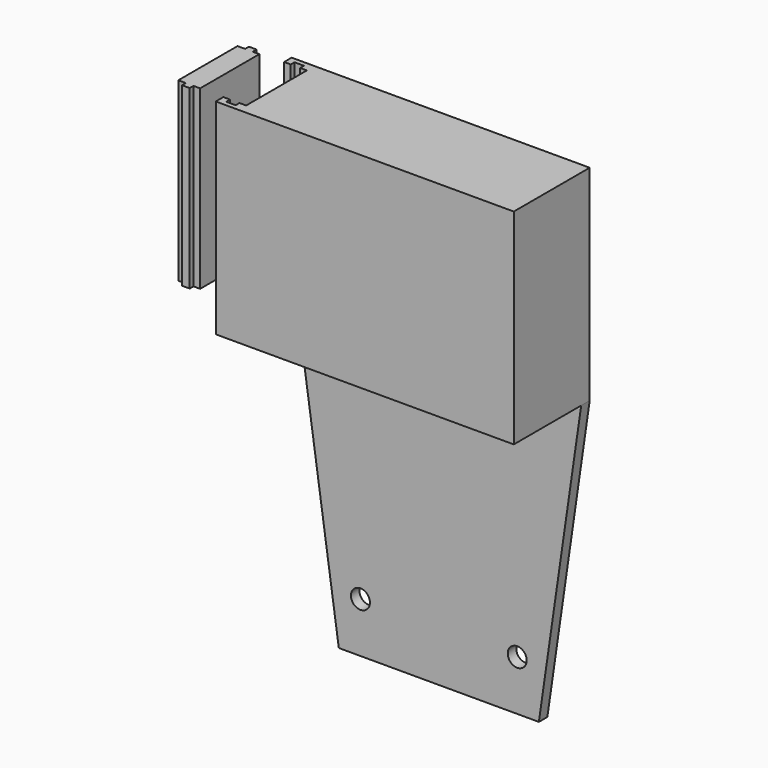
from build123d import *

# Parameters (mm, degrees)
F0_W      = 70
F0_H      = 49
F0_W_2    = 26.35
F0_H_2    = 0.8
F0_R      = 2.5
F0_W_3    = 3.5
F0_H_3    = 2.5
F0_W_4    = 2.5
F1_DEPTH  = 25
F2_DEPTH  = 22.5
F3_DEPTH  = 2.5
F6_W      = 2.5
F6_H      = 1.25
F7_DEPTH  = 51.5
F8_DEPTH  = 47.5
F9_DEPTH  = 46.5
F10_DEPTH = 22.2


# Not quite as in the source:
# - a feature names something its author has since deleted; it is built from what else it names


with BuildPart() as f1:
    # F0 (on Front) → F1 (new body)
    with BuildSketch(Plane.XZ):
        Polygon((-35, 24), (35, 24), (35, -25), (-35, -25), (-35, -27.5), (-26.35, -27.5), (0, -27.5), (26.35, -27.5), (37.5, -27.5), (37.5, 26.5), (-35, 26.5), align=None)
        with Locations((0, -0.5)):
            Rectangle(F0_W, F0_H)
        Polygon((26.35, -104.5), (37.5, -27.5), (26.35, -27.5), (26.35, -28.3), align=None)
        with Locations((-13.175, -27.9)):
            Rectangle(F0_W_2, F0_H_2)
        with Locations((13.175, -27.9)):
            Rectangle(F0_W_2, F0_H_2)
        Polygon((0, -28.3), (-26.35, -28.3), (-26.35, -104.5), (26.35, -104.5), (26.35, -28.3), align=None)
        with Locations((-20.65, -91.3)):
            Circle(F0_R, mode=Mode.SUBTRACT)
        with Locations((20.65, -91.3)):
            Circle(F0_R, mode=Mode.SUBTRACT)
        with Locations((-20.65, -37.3)):
            Circle(F0_R, mode=Mode.SUBTRACT)
        with Locations((20.65, -37.3)):
            Circle(F0_R, mode=Mode.SUBTRACT)
        Polygon((-26.35, -27.5), (-35, -27.5), (-37.5, -27.5), (-26.35, -104.5), (-26.35, -28.3), align=None)
        with Locations((-39.25, -26.25)):
            Rectangle(F0_W_3, F0_H_3)
        with Locations((-36.25, -26.25)):
            Rectangle(F0_W_4, F0_H_3)
    extrude(amount=-F1_DEPTH)

    # F0 (on Front) → F2 (cut)
    with BuildSketch(Plane.XZ):
        with Locations((0, -0.5)):
            Rectangle(F0_W, F0_H)
    extrude(amount=-F2_DEPTH, mode=Mode.SUBTRACT)

    # F0 (on Front) → F3 (join)
    with BuildSketch(Plane.XZ):
        with Locations((0, -0.5)):
            Rectangle(F0_W, F0_H)
    extrude(amount=-F3_DEPTH)

    # F6 (on 3pt) → F7 (join)
    with BuildSketch(Plane(origin=(0, 0, 26.5), x_dir=(1, 0, 0), z_dir=(0, 0, -1))):
        Polygon((-35, -25), (-35, -22.5), (-36.75, -22.5), (-36.75, -23.75), (-39.25, -23.75), (-39.25, -22.5), (-41, -22.5), (-41, -25), align=None)
        Polygon((-35, -2.5), (-35, 0), (-41, 0), (-41, -2.5), (-39.25, -2.5), (-39.25, -1.25), (-36.75, -1.25), (-36.75, -2.5), align=None)
        with Locations((-38, -1.875)):
            Rectangle(F6_W, F6_H)
        with Locations((-38, -23.125)):
            Rectangle(F6_W, F6_H)
    extrude(amount=F7_DEPTH)

    # F6 (on 3pt) → F8 (cut)
    with BuildSketch(Plane(origin=(0, 0, 26.5), x_dir=(1, 0, 0), z_dir=(0, 0, -1))):
        with Locations((-38, -23.125)):
            Rectangle(F6_W, F6_H)
        with Locations((-38, -1.875)):
            Rectangle(F6_W, F6_H)
    extrude(amount=F8_DEPTH, mode=Mode.SUBTRACT)

    # F0 (on Front) → F10 (cut)
    with BuildSketch(Plane.XZ):
        Polygon((-26.35, -27.5), (-35, -27.5), (-37.5, -27.5), (-26.35, -104.5), (-26.35, -28.3), align=None)
        Polygon((0, -28.3), (-26.35, -28.3), (-26.35, -104.5), (26.35, -104.5), (26.35, -28.3), align=None)
        with Locations((-20.65, -91.3)):
            Circle(F0_R, mode=Mode.SUBTRACT)
        with Locations((20.65, -91.3)):
            Circle(F0_R, mode=Mode.SUBTRACT)
        with Locations((-20.65, -37.3)):
            Circle(F0_R, mode=Mode.SUBTRACT)
        with Locations((20.65, -37.3)):
            Circle(F0_R, mode=Mode.SUBTRACT)
        Polygon((26.35, -104.5), (37.5, -27.5), (26.35, -27.5), (26.35, -28.3), align=None)
        with Locations((-13.175, -27.9)):
            Rectangle(F0_W_2, F0_H_2)
        with Locations((13.175, -27.9)):
            Rectangle(F0_W_2, F0_H_2)
    extrude(amount=-F10_DEPTH, mode=Mode.SUBTRACT)


with BuildPart() as f9:
    # F6 (on 3pt) → F9 (new body)
    with BuildSketch(Plane(origin=(0, 0, 26.5), x_dir=(1, 0, 0), z_dir=(0, 0, -1))):
        Polygon((-52.9117025435, -2.5576207936), (-52.9117025435, -22.0576207936), (-50.9117025435, -22.0576207936), (-50.9117025435, -23.3076207936), (-48.9117025435, -23.3076207936), (-48.9117025435, -22.0576207936), (-47.1617025435, -22.0576207936), (-47.1617025435, -2.5576207936), (-48.9117025435, -2.5576207936), (-48.9117025435, -1.3076207936), (-50.9117025435, -1.3076207936), (-50.9117025435, -2.5576207936), align=None)
    extrude(amount=F9_DEPTH)


solid = Compound([f1.part, f9.part])
